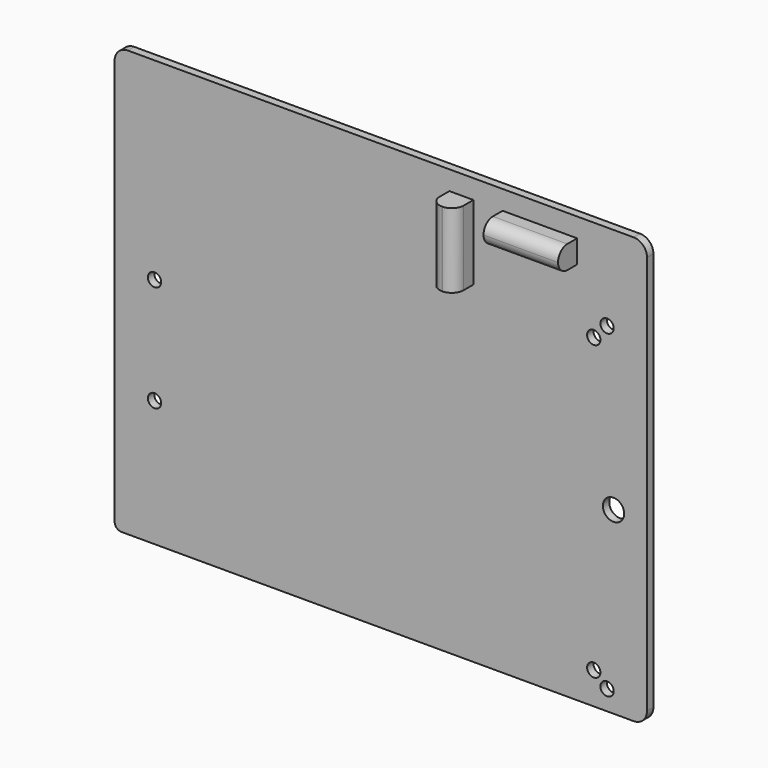
from build123d import *

# Parameters (mm, degrees)
F0_R        = 3.175
F0_W        = 11.43
F0_H        = 35.56
F0_W_2      = 35.56
F0_H_2      = 10.9884785938
F1_DEPTH    = 3.81
F2_DEPTH    = 15.24
F3_T1_DEPTH = 35.56
F3_T3_DEPTH = 35.56


# Not quite as in the source:
# - a fillet or chamfer that OpenCascade refuses, or shapes differently, is made with other operations: its cross-section is extruded or revolved along the edge and cut away or added


with BuildPart() as f1:
    # F0 (on Front) → F1 (new body)
    with BuildSketch(Plane.XZ):
        with BuildLine():
            Line((246.8790987015, 3.8439502823), (5.5790987015, 3.8439502823))
            ThreePointArc((5.5790987015, 3.8439502823), (1.0889706409, 1.9840783429), (-0.7709012985, -2.5060497177))
            Line((-0.7709012985, -2.5060497177), (-0.7709012985, -196.0790987015))
            ThreePointArc((-0.7709012985, -196.0790987015), (0.1888954325, -198.3962529867), (2.5060497177, -199.3560497177))
            Line((2.5060497177, -199.3560497177), (246.8790987015, -199.3560497177))
            ThreePointArc((246.8790987015, -199.3560497177), (251.369226762, -197.4961777782), (253.2290987015, -193.0060497177))
            Line((253.2290987015, -193.0060497177), (253.2290987015, -2.5060497177))
            ThreePointArc((253.2290987015, -2.5060497177), (251.369226762, 1.9840783429), (246.8790987015, 3.8439502823))
        make_face()
        with Locations((18.2790987015, -139.0930234075)):
            Circle(F0_R, mode=Mode.SUBTRACT)
        with Locations((234.1790987015, -189.8930234075)):
            Circle(F0_R, mode=Mode.SUBTRACT)
        with Locations((227.8290987015, -184.0757250905)):
            Circle(F0_R, mode=Mode.SUBTRACT)
        with BuildLine():
            ThreePointArc((232.1718121719, -113.6930234075), (237.2518121719, -108.6130234075), (242.3318121719, -113.6930234075))
            ThreePointArc((242.3318121719, -113.6930234075), (237.2518121719, -118.7730234075), (232.1718121719, -113.6930234075))
        make_face(mode=Mode.SUBTRACT)
        with Locations((18.2790987015, -88.2930234075)):
            Circle(F0_R, mode=Mode.SUBTRACT)
        with Locations((164.6692329311, -23.1037478608)):
            Rectangle(F0_W, F0_H, mode=Mode.SUBTRACT)
        with Locations((227.8290987015, -44.3757250905)):
            Circle(F0_R, mode=Mode.SUBTRACT)
        with Locations((234.1790987015, -37.4930234075)):
            Circle(F0_R, mode=Mode.SUBTRACT)
        with Locations((202.1326256323, -10.8179871577)):
            Rectangle(F0_W_2, F0_H_2, mode=Mode.SUBTRACT)
        with Locations((164.6692329311, -23.1037478608)):
            Rectangle(F0_W, F0_H)
        with Locations((202.1326256323, -10.8179871577)):
            Rectangle(F0_W_2, F0_H_2)
    extrude(amount=F1_DEPTH)

    # F0 (on Front) → F2 (join)
    with BuildSketch(Plane.XZ):
        with Locations((164.6692329311, -23.1037478608)):
            Rectangle(F0_W, F0_H)
        with Locations((202.1326256323, -10.8179871577)):
            Rectangle(F0_W_2, F0_H_2)
    extrude(amount=F2_DEPTH)

    # F3: fillet of radius 5.588 on 4 edges, made by hand

    # F3_s2 → F3_t1 (cut)
    with BuildSketch(Plane.XY.offset(-40.8837478608)):
        with BuildLine():
            ThreePointArc((158.9542329311, -9.652), (160.5909202379, -13.6033126933), (164.5422329311, -15.24))
            Line((164.5422329311, -15.24), (164.5422329311, -15.35176))
            Line((164.5422329311, -15.35176), (158.8424729311, -15.35176))
            Line((158.8424729311, -15.35176), (158.8424729311, -9.652))
            Line((158.8424729311, -9.652), (158.9542329311, -9.652))
        make_face()
        with BuildLine():
            ThreePointArc((170.3842329311, -9.652), (168.7475456244, -13.6033126933), (164.7962329311, -15.24))
            Line((164.7962329311, -15.24), (164.7962329311, -15.35176))
            Line((164.7962329311, -15.35176), (170.4959929311, -15.35176))
            Line((170.4959929311, -15.35176), (170.4959929311, -9.652))
            Line((170.4959929311, -9.652), (170.3842329311, -9.652))
        make_face()
    extrude(amount=F3_T1_DEPTH, mode=Mode.SUBTRACT)

    # F3_s4 → F3_t3 (cut)
    with BuildSketch(Plane.YZ.offset(184.3526256323)):
        with BuildLine():
            ThreePointArc((-9.652, -5.3237478608), (-13.6033126933, -6.9604351675), (-15.24, -10.9117478608))
            Line((-15.24, -10.9117478608), (-15.35176, -10.9117478608))
            Line((-15.35176, -10.9117478608), (-15.35176, -5.2119878608))
            Line((-15.35176, -5.2119878608), (-9.652, -5.2119878608))
            Line((-9.652, -5.2119878608), (-9.652, -5.3237478608))
        make_face()
        with BuildLine():
            ThreePointArc((-9.652, -16.3122264546), (-13.6033126933, -14.6755391479), (-15.24, -10.7242264546))
            Line((-15.24, -10.7242264546), (-15.35176, -10.7242264546))
            Line((-15.35176, -10.7242264546), (-15.35176, -16.4239864546))
            Line((-15.35176, -16.4239864546), (-9.652, -16.4239864546))
            Line((-9.652, -16.4239864546), (-9.652, -16.3122264546))
        make_face()
    extrude(amount=F3_T3_DEPTH, mode=Mode.SUBTRACT)


solid = f1.part
